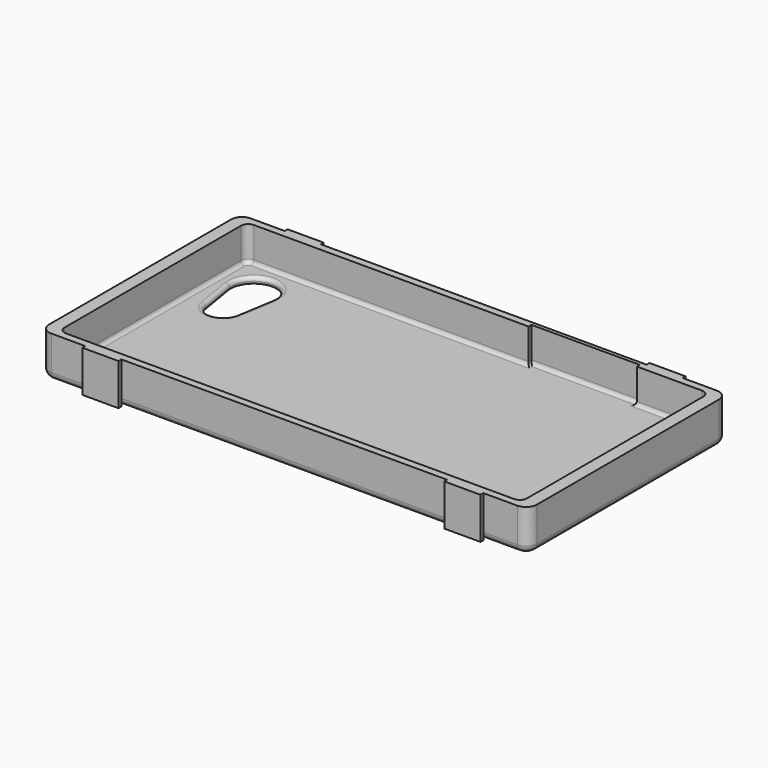
from build123d import *

# Parameters (mm, degrees)
F0_W         = 135
F0_H         = 69
F1_DEPTH     = 11.5
F2_DEPTH     = 2
F3_R         = 2
F4_R         = 2
F5_R         = 1
F6_T1_DEPTH  = 19
F6_T4_ANGLE  = 90
F6_T6_ANGLE  = 90
F6_T8_ANGLE  = 90
F6_T10_ANGLE = 90
F7_W         = 10
F7_H         = 1
F8_DEPTH     = 11.5
F10_DEPTH    = 25
F11_R        = 0.99999


# Not quite as in the source:
# - a fillet or chamfer that OpenCascade refuses, or shapes differently, is made with other operations: its cross-section is extruded or revolved along the edge and cut away or added
# - a fillet or chamfer is up to 0.001 mm smaller than in the source, because OpenCascade refuses the exact size
# - a feature of the source that left no trace in its solid (it failed there, or was rolled back) is left out


with BuildPart() as f1:
    # F0 (on Top) → F1 (new body)
    with BuildSketch(Plane.XY):
        Rectangle(F0_W, F0_H)
        Polygon((-64, -32.5), (-64, 32.5), (14, 32.5), (14, 33.5), (44, 33.5), (44, 32.5), (64, 32.5), (64, -32.5), align=None, mode=Mode.SUBTRACT)
    extrude(amount=F1_DEPTH)

    # F0 (on Top) → F2 (join)
    with BuildSketch(Plane.XY):
        Polygon((14, 32.5), (-64, 32.5), (-64, -32.5), (64, -32.5), (64, 32.5), (44, 32.5), (44, 33.5), (14, 33.5), align=None)
    extrude(amount=F2_DEPTH)

    # F3
    f3_edges = [f1.edges().sort_by_distance(p)[0] for p in [
        (0, 34.5, 0),
        (-67.5, 0, 0),
        (0, -34.5, 0),
        (67.5, 0, 0),
    ]]
    fillet(f3_edges, radius=F3_R)

    # F4
    f4_edges = [f1.edges().sort_by_distance(p)[0] for p in [
        (-64, 32.5, 6.75),
        (64, 32.5, 6.75),
        (64, -32.5, 6.75),
        (-64, -32.5, 6.75),
    ]]
    fillet(f4_edges, radius=F4_R)

    # F5
    f5_edges = [f1.edges().sort_by_distance(p)[0] for p in [
        (-24, 32.5, 2),
        (-63.414214, 31.914214, 2),
        (14, 33, 2),
        (-64, 0, 2),
        (29, 33.5, 2),
        (-63.414214, -31.914214, 2),
        (44, 33, 2),
        (0, -32.5, 2),
        (53, 32.5, 2),
        (63.414214, -31.914214, 2),
        (63.414214, 31.914214, 2),
        (64, 0, 2),
    ]]
    fillet(f5_edges, radius=F5_R)

    # F6: fillet of radius 3 on 4 edges, made by hand

    # F6_s2 → F6_t1 (cut)
    with BuildSketch(Plane.XY):
        with BuildLine():
            ThreePointArc((-64.5, 34.5), (-66.6213203436, 33.6213203436), (-67.5, 31.5))
            Line((-67.5, 31.5), (-67.5, 34.5))
            Line((-67.5, 34.5), (-64.5, 34.5))
        make_face()
        with BuildLine():
            ThreePointArc((-67.5, -31.5), (-66.6213203436, -33.6213203436), (-64.5, -34.5))
            Line((-64.5, -34.5), (-67.5, -34.5))
            Line((-67.5, -34.5), (-67.5, -31.5))
        make_face()
        with BuildLine():
            ThreePointArc((64.5, -34.5), (66.6213203436, -33.6213203436), (67.5, -31.5))
            Line((67.5, -31.5), (67.5, -34.5))
            Line((67.5, -34.5), (64.5, -34.5))
        make_face()
        with BuildLine():
            ThreePointArc((64.5, 34.5), (66.6213203436, 33.6213203436), (67.5, 31.5))
            Line((67.5, 31.5), (67.5, 34.5))
            Line((67.5, 34.5), (64.5, 34.5))
        make_face()
    extrude(amount=F6_T1_DEPTH, mode=Mode.SUBTRACT)

    # F6_s3 → F6_t4 (revolve, cut)
    with BuildSketch(Plane.YZ.offset(64.5)):
        with BuildLine():
            ThreePointArc((32.5, 0), (33.9142135624, 0.5857864376), (34.5, 2))
            Line((34.5, 2), (34.5, 0))
            Line((34.5, 0), (32.5, 0))
        make_face()
    revolve(axis=Axis((64.5, 31.5, 0), (0, 0, -1)), revolution_arc=F6_T4_ANGLE, mode=Mode.SUBTRACT)

    # F6_s5 → F6_t6 (revolve, cut)
    with BuildSketch(Plane.XZ.offset(31.5)):
        with BuildLine():
            ThreePointArc((65.5, 0), (66.9142135624, 0.5857864376), (67.5, 2))
            Line((67.5, 2), (67.5, 0))
            Line((67.5, 0), (65.5, 0))
        make_face()
    revolve(axis=Axis((64.5, -31.5, 0), (0, 0, -1)), revolution_arc=F6_T6_ANGLE, mode=Mode.SUBTRACT)

    # F6_s7 → F6_t8 (revolve, cut)
    with BuildSketch(Plane.YZ.offset(-64.5)):
        with BuildLine():
            ThreePointArc((-32.5, 0), (-33.9142135624, 0.5857864376), (-34.5, 2))
            Line((-34.5, 2), (-34.5, 0))
            Line((-34.5, 0), (-32.5, 0))
        make_face()
    revolve(axis=Axis((-64.5, -31.5, 0), (0, 0, -1)), revolution_arc=F6_T8_ANGLE, mode=Mode.SUBTRACT)

    # F6_s9 → F6_t10 (revolve, cut)
    with BuildSketch(Plane.XZ.offset(-31.5)):
        with BuildLine():
            ThreePointArc((-65.5, 0), (-66.9142135624, 0.5857864376), (-67.5, 2))
            Line((-67.5, 2), (-67.5, 0))
            Line((-67.5, 0), (-65.5, 0))
        make_face()
    revolve(axis=Axis((-64.5, 31.5, 0), (0, 0, -1)), revolution_arc=F6_T10_ANGLE, mode=Mode.SUBTRACT)

    # F7 (on face) → F8 (join, through all)
    with BuildSketch(Plane.XY.offset(11.5)):
        with Locations((-50.1, 35)):
            Rectangle(F7_W, F7_H)
        with Locations((50.1, 35)):
            Rectangle(F7_W, F7_H)
        with Locations((-50.1, -35)):
            Rectangle(F7_W, F7_H)
        with Locations((50.1, -35)):
            Rectangle(F7_W, F7_H)
    extrude(amount=-F8_DEPTH)

    # F9 (on face) → F10 (cut)
    with BuildSketch(Plane.XY.offset(2)):
        with BuildLine():
            Line((-50.2595349939, 11.8031518124), (-48.5794111489, 22.0270520794))
            ThreePointArc((-48.5794111489, 22.0270520794), (-54.5, 29), (-60.4205888511, 22.0270520794))
            Line((-60.4205888511, 22.0270520794), (-58.7404650061, 11.8031518124))
            ThreePointArc((-58.7404650061, 11.8031518124), (-54.5, 8.2026588611), (-50.2595349939, 11.8031518124))
        make_face()
    extrude(amount=-F10_DEPTH, mode=Mode.SUBTRACT)

    # F11 (radius 1 in the source; OpenCascade refuses exactly that, so slightly less here)
    f11_edges = [f1.edges().sort_by_distance(p)[0] for p in [
        (-54.5, 29, 2),
        (-49.419473, 16.915102, 0),
        (-54.5, 8.202659, 2),
        (-49.419473, 16.915102, 2),
        (-59.580527, 16.915102, 2),
        (-54.5, 8.202659, 0),
        (-54.5, 29, 0),
        (-59.580527, 16.915102, 0),
    ]]
    fillet(f11_edges, radius=F11_R)


solid = f1.part
